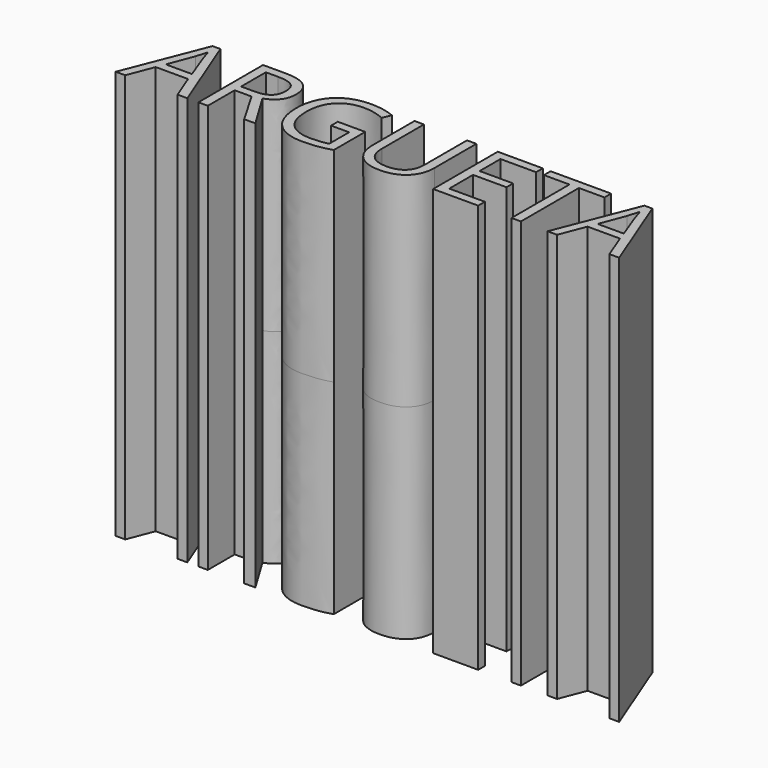
from build123d import *

# Parameters (mm, degrees)
F0_TEXT_SIZE = 14.0676382014
F1_DEPTH     = 25.4


# Not quite as in the source:
# - Text() gives the source's letters only with a copy of the font that has no kerning and outlines rounded to 1/6400 em; it was checked with that copy


with BuildPart() as f1:
    # F0 (on Top) → F1 (new body, symmetric)
    with BuildSketch(Plane.XY):
        with Locations((-28.8251689145, -4.8215384336)):
            Text('ARGUETA', F0_TEXT_SIZE, font='Open Sans', text_align=(TextAlign.LEFT, TextAlign.BOTTOM))
    extrude(amount=F1_DEPTH, both=True)


solid = f1.part
